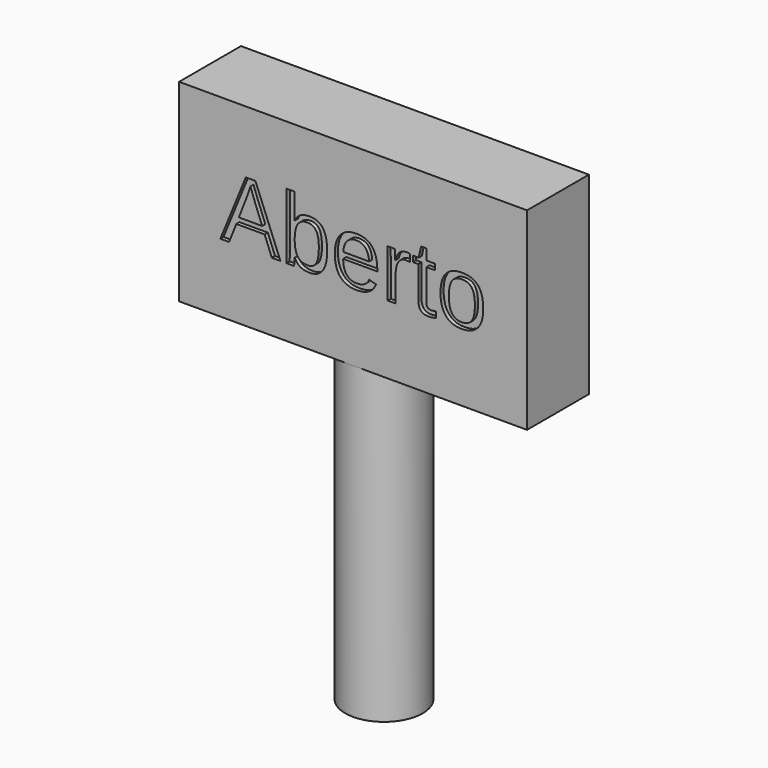
from build123d import *

# Parameters (mm, degrees)
F0_W         = 45
F0_H         = 25
F1_DEPTH     = 10
F2_TEXT_SIZE = 11.7145192391
F3_DEPTH     = 0.508
F4_TEXT_SIZE = 10.292271774
F5_DEPTH     = 0.508
F6_R         = 5
F7_DEPTH     = 40
F8_R         = 2.5
F9_DEPTH     = 7


# Not quite as in the source:
# - Text() gives the source's letters only with a copy of the font that has no kerning and outlines rounded to 1/6400 em; it was checked with that copy


with BuildPart() as f1:
    # F0 (on Front) → F1 (new body)
    with BuildSketch(Plane.XZ):
        with Locations((-23.8699549437, -21.8419387937)):
            Rectangle(F0_W, F0_H)
    extrude(amount=F1_DEPTH)

    # F2 (on face) → F3 (cut)
    with BuildSketch(Plane.XZ.offset(10)):
        with Locations((-41.055809758, -25.4792195386)):
            Text('Aberto', F2_TEXT_SIZE, font='Arimo', text_align=(TextAlign.LEFT, TextAlign.BOTTOM))
    extrude(amount=-F3_DEPTH, mode=Mode.SUBTRACT)

    # F4 (on face) → F5 (cut)
    with BuildSketch(Plane(origin=(0, 0, 0), x_dir=(-1, 0, 0), z_dir=(0, 1, 0))):
        with Locations((3.5455549437, -25.5407744709)):
            Text('Fechado', F4_TEXT_SIZE, font='Open Sans', text_align=(TextAlign.LEFT, TextAlign.BOTTOM))
    extrude(amount=-F5_DEPTH, mode=Mode.SUBTRACT)

    # F6 (on face) → F7 (join)
    with BuildSketch(Plane(origin=(0, 0, -34.3419387937), x_dir=(1, 0, 0), z_dir=(0, 0, -1))):
        with Locations((-23.8705549437, 5)):
            Circle(F6_R)
    extrude(amount=F7_DEPTH)

    # F8 (on face) → F9 (cut)
    with BuildSketch(Plane(origin=(0, 0, -74.3419387937), x_dir=(1, 0, 0), z_dir=(0, 0, -1))):
        with Locations((-23.8705549437, 5)):
            Circle(F8_R)
    extrude(amount=-F9_DEPTH, mode=Mode.SUBTRACT)


solid = f1.part
